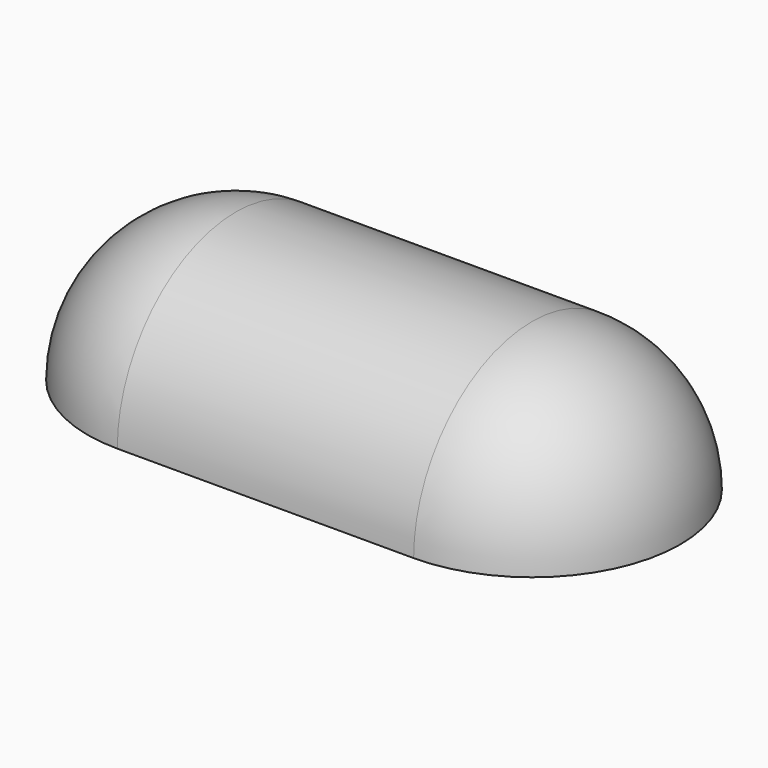
from build123d import *

# Parameters (mm, degrees)
F1_ANGLE = 180
F3_ANGLE = 180
F5_ANGLE = 180


with BuildPart() as f1:
    # F0 (on Top) → F1 (revolve)
    with BuildSketch(Plane.XY):
        Polygon((22.25, -22.25), (22.25, 0), (17.25, 0), (17.25, -17.25), (-17.25, -17.25), (-17.25, 0), (-22.25, 0), (-22.25, -22.25), align=None)
    revolve(axis=Axis((4.6253763139, 0, 0), (-1, 0, 0)), revolution_arc=F1_ANGLE)

    # F2 (on face) → F3 (revolve)
    with BuildSketch(Plane.YZ.offset(22.25)):
        with BuildLine():
            ThreePointArc((0, 22.25), (-15.7331258814, 15.7331258814), (-22.25, 0))
            Line((-22.25, 0), (-17.25, 0))
            ThreePointArc((-17.25, 0), (-12.1975919755, 12.1975919755), (0, 17.25))
            Line((0, 17.25), (0, 22.25))
        make_face()
    revolve(axis=Axis((22.25, 0, 10.080948472), (0, 0, 1)), revolution_arc=F3_ANGLE)

    # F4 (on face) → F5 (revolve)
    with BuildSketch(Plane(origin=(-22.25, 0, 0), x_dir=(0, -1, 0), z_dir=(-1, 0, 0))):
        with BuildLine():
            ThreePointArc((0, 22.25), (-15.7331258814, 15.7331258814), (-22.25, 0))
            Line((-22.25, 0), (-17.6879018545, 0))
            ThreePointArc((-17.6879018545, 0), (-12.5072353463, 12.5072353463), (0, 17.6879018545))
            Line((0, 17.6879018545), (0, 22.25))
        make_face()
    revolve(axis=Axis((-22.25, 0, 6.120197475), (0, 0, 1)), revolution_arc=F5_ANGLE)


solid = f1.part
